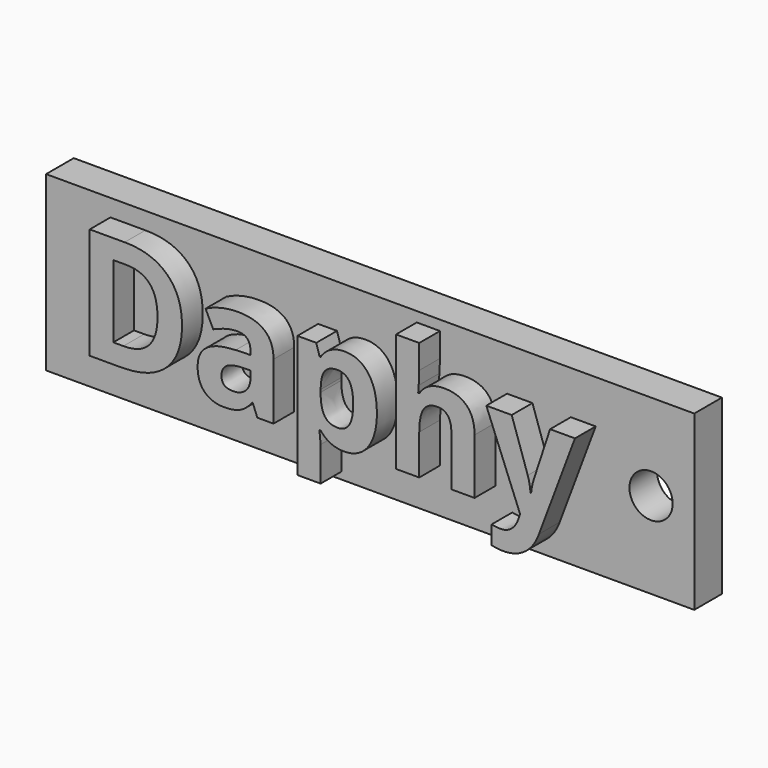
from build123d import *

# Parameters (mm, degrees)
F0_W         = 75
F0_H         = 20
F0_R         = 2.5
F1_DEPTH     = 4
F2_TEXT_SIZE = 18.0341406829
F3_DEPTH     = 3


# Not quite as in the source:
# - Text() gives the source's letters only with a copy of the font that has no kerning and outlines rounded to 1/6400 em; it was checked with that copy


with BuildPart() as f1:
    # F0 (on Front) → F1 (new body)
    with BuildSketch(Plane.XZ):
        with Locations((37.5, -10)):
            Rectangle(F0_W, F0_H)
        with Locations((70, -10)):
            Circle(F0_R, mode=Mode.SUBTRACT)
    extrude(amount=F1_DEPTH)

    # F2 (on face) → F3 (join)
    with BuildSketch(Plane.XZ.offset(4)):
        with Locations((5.8271065354, -14.8651860654)):
            Text('Daphy', F2_TEXT_SIZE, font='Open Sans', font_style=FontStyle.BOLD, text_align=(TextAlign.LEFT, TextAlign.BOTTOM))
    extrude(amount=F3_DEPTH)


solid = f1.part
